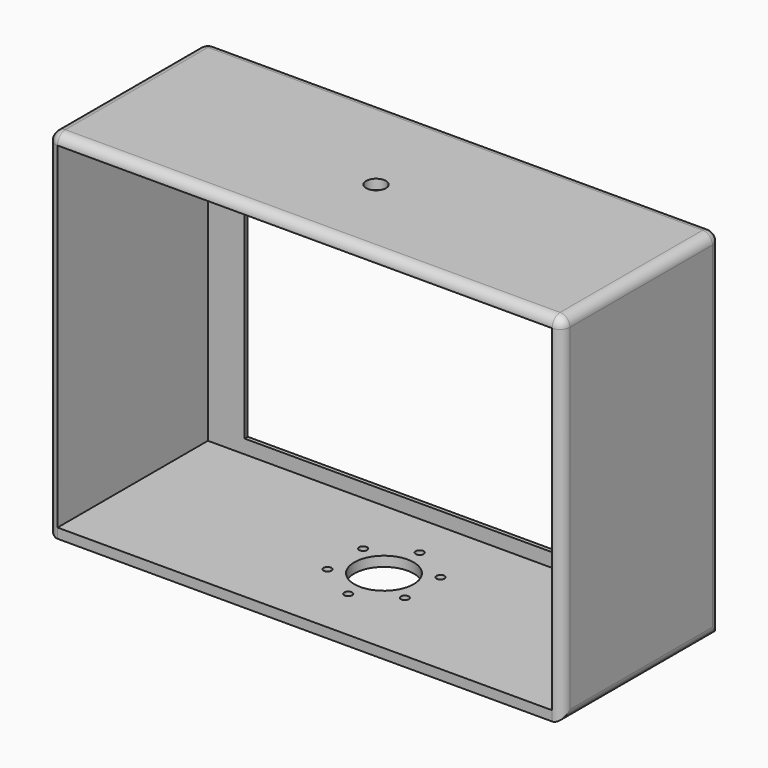
from build123d import *

# Parameters (mm, degrees)
F0_W      = 260
F0_H      = 100
F1_DEPTH  = 180
F2_T      = -5
F3_W      = 223
F3_H      = 143
F3_W_2    = 212.9999995232
F3_H_2    = 132.9999995232
F4_DEPTH  = 3
F5_DEPTH  = 25
F3_R      = 4.5
F6_DEPTH  = 25
F7_R      = 2
F7_R_2    = 15
F8_DEPTH  = 25
F9_R      = 4.99999
F10_R     = 5
F11_DEPTH = 25


# Not quite as in the source:
# - a fillet or chamfer is up to 0.001 mm smaller than in the source, because OpenCascade refuses the exact size


with BuildPart() as f1:
    # F0 (on Top) → F1 (new body)
    with BuildSketch(Plane.XY):
        Rectangle(F0_W, F0_H)
    extrude(amount=F1_DEPTH)

    # F2
    f2_openings = [f1.faces().sort_by_distance(p)[0] for p in [
        (0, -50, 90),
    ]]
    offset(amount=F2_T, openings=f2_openings)

    # F3 (on face) → F4 (cut)
    with BuildSketch(Plane(origin=(0, 50, 0), x_dir=(-1, 0, 0), z_dir=(0, 1, 0))):
        with Locations((0, 78.5)):
            Rectangle(F3_W, F3_H)
        with Locations((0, 78.5)):
            Rectangle(F3_W_2, F3_H_2, mode=Mode.SUBTRACT)
    extrude(amount=-F4_DEPTH, mode=Mode.SUBTRACT)

    # F5 (cut): a face of the model
    f5_faces = [f1.faces().sort_by_distance(p)[0] for p in [
        (0, 50, 78.5),
    ]]
    extrude(f5_faces, amount=-F5_DEPTH, mode=Mode.SUBTRACT)

    # F3 (on face) → F6 (cut)
    with BuildSketch(Plane(origin=(0, 50, 0), x_dir=(-1, 0, 0), z_dir=(0, 1, 0))):
        with Locations((-45, 163)):
            Circle(F3_R)
        with Locations((45, 163)):
            Circle(F3_R)
    extrude(amount=-F6_DEPTH, mode=Mode.SUBTRACT)

    # F7 (on face) → F8 (cut)
    with BuildSketch(Plane(origin=(0, 0, 0), x_dir=(1, 0, 0), z_dir=(0, 0, -1))):
        with Locations((-19.5557196429, 11.2905)):
            Circle(F7_R)
        with Locations((0, 22.581)):
            Circle(F7_R)
        with Locations((19.5557196429, 11.2905)):
            Circle(F7_R)
        with Locations((19.5557196429, -11.2905)):
            Circle(F7_R)
        with Locations((0, -22.581)):
            Circle(F7_R)
        with Locations((-19.5557196429, -11.2905)):
            Circle(F7_R)
        Circle(F7_R_2)
    extrude(amount=-F8_DEPTH, mode=Mode.SUBTRACT)

    # F9 (radius 5 in the source; OpenCascade refuses exactly that, so slightly less here)
    f9_edges = [f1.edges().sort_by_distance(p)[0] for p in [
        (0, 50, 180),
        (-130, 0, 180),
        (-130, 50, 90),
        (-130, -50, 90),
        (-130, 0, 0),
        (0, -50, 180),
        (130, 0, 180),
        (130, -50, 90),
        (130, 50, 90),
        (130, 0, 0),
    ]]
    fillet(f9_edges, radius=F9_R)

    # F10 (on face) → F11 (cut)
    with BuildSketch(Plane.XY.offset(180)):
        with Locations((0, -5)):
            Circle(F10_R)
    extrude(amount=-F11_DEPTH, mode=Mode.SUBTRACT)


solid = f1.part
